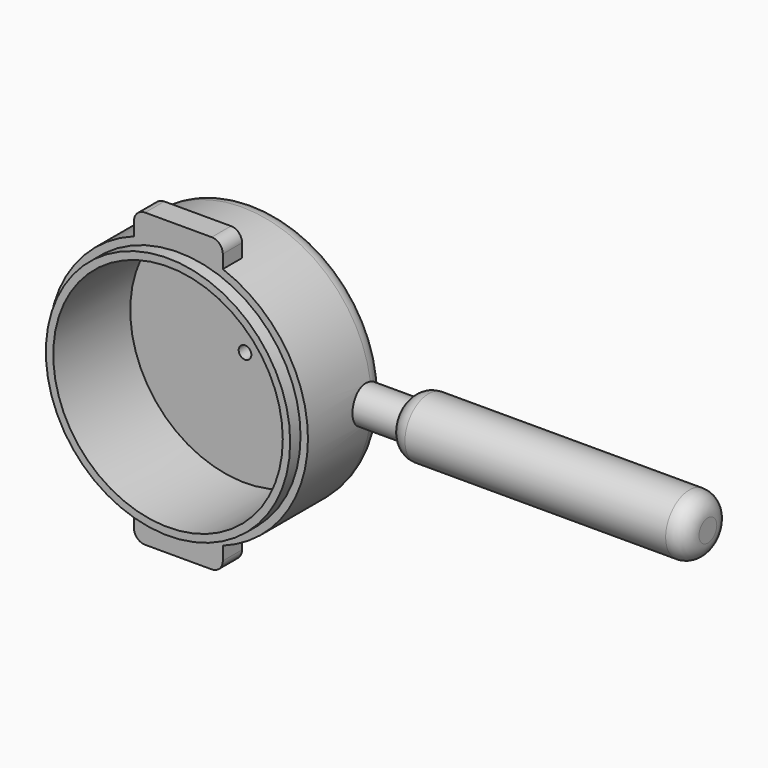
from build123d import *

# Parameters (mm, degrees)
F0_R      = 35
F1_DEPTH  = 30
F2_T      = -4
F3_R      = 5
F5_R      = 5
F7_R      = 8
F7_R_2    = 5
F8_DEPTH  = 80
F9_R      = 5.0065220345
F10_DEPTH = 7
F11_SIZE  = 2
F14_DEPTH = 6.5
F15_R     = 5
F17_R     = 35
F17_R_2   = 33
F18_DEPTH = 3.5
F19_R     = 3
F20_R     = 1.7097163671
F21_DEPTH = 37.001


# Not quite as in the source:
# - a fillet or chamfer that OpenCascade refuses, or shapes differently, is made with other operations: its cross-section is extruded or revolved along the edge and cut away or added


with BuildPart() as f1:
    # F0 (on Front) → F1 (new body)
    with BuildSketch(Plane.XZ):
        Circle(F0_R)
    extrude(amount=F1_DEPTH)

    # F2
    f2_openings = [f1.faces().sort_by_distance(p)[0] for p in [
        (0, -30, 0),
    ]]
    offset(amount=F2_T, openings=f2_openings)

    # F3
    f3_edges = [f1.edges().sort_by_distance(p)[0] for p in [
        (-35, 0, 0),
    ]]
    fillet(f3_edges, radius=F3_R)

    # F5 (on offset) → F6 (join, up to the next surface of F1)
    with BuildSketch(Plane.YZ.offset(47)):
        with Locations((-6.4707305679, 0)):
            Circle(F5_R)
    extrude(until=Until.NEXT, dir=(-1, 0, 0))

    # F7 (on face) → F8 (join)
    with BuildSketch(Plane.YZ.offset(47)):
        with Locations((-6.4707305679, 0)):
            Circle(F7_R)
        with Locations((-6.4707305679, 0)):
            Circle(F7_R_2, mode=Mode.SUBTRACT)
        with Locations((-6.4707305679, 0)):
            Circle(F7_R_2)
    extrude(amount=F8_DEPTH)

    # F9 (on face) → F10 (join)
    with BuildSketch(Plane(origin=(0, 0, 0), x_dir=(-1, 0, 0), z_dir=(0, 1, 0))):
        Circle(F9_R)
    extrude(amount=F10_DEPTH)

    # F11
    f11_edges = [f1.edges().sort_by_distance(p)[0] for p in [
        (5.006522, 7, 0),
    ]]
    chamfer(f11_edges, length=F11_SIZE)

    # F13 (on offset) → F14 (join)
    with BuildSketch(Plane.XZ.offset(26.5)):
        with BuildLine():
            Line((-12, -39.5), (12, -39.5))
            Line((12, -39.5), (12, -32.8785644455))
            ThreePointArc((12, -32.8785644455), (0, -35), (-12, -32.8785644455))
            Line((-12, -32.8785644455), (-12, -39.5))
        make_face()
        with BuildLine():
            ThreePointArc((-12, 32.8785644455), (0, 35), (12, 32.8785644455))
            Line((12, 32.8785644455), (12, 39.5))
            Line((12, 39.5), (-12, 39.5))
            Line((-12, 39.5), (-12, 32.8785644455))
        make_face()
    extrude(amount=-F14_DEPTH)

    # F15
    f15_edges = [f1.edges().sort_by_distance(p)[0] for p in [
        (127, -14.470731, 0),
    ]]
    fillet(f15_edges, radius=F15_R)

    # F16: fillet of radius 5 on 1 edges, made by hand

    # F16_s1 → F16_t2 (revolve, cut)
    with BuildSketch(Plane.XY):
        with BuildLine():
            ThreePointArc((51.582575695, 1.5292694321), (48.8439629074, 0.7125695648), (47, -1.4707305679))
            Line((47, -1.4707305679), (47, 1.5292694321))
            Line((47, 1.5292694321), (51.582575695, 1.5292694321))
        make_face()
    revolve(axis=Axis((47, -6.4707305679, 0), (1, 0, 0)), mode=Mode.SUBTRACT)

    # F17 (on face) → F18 (cut, through all)
    with BuildSketch(Plane.XZ.offset(30)):
        Circle(F17_R)
        Circle(F17_R_2, mode=Mode.SUBTRACT)
    extrude(amount=-F18_DEPTH, mode=Mode.SUBTRACT)

    # F19
    f19_edges = [f1.edges().sort_by_distance(p)[0] for p in [
        (12, -23.25, 39.5),
        (-12, -23.25, 39.5),
        (-12, -23.25, -39.5),
        (12, -23.25, -39.5),
    ]]
    fillet(f19_edges, radius=F19_R)

    # F20 (on face) → F21 (cut, through all)
    with BuildSketch(Plane(origin=(0, 7, 0), x_dir=(-1, 0, 0), z_dir=(0, 1, 0))):
        Circle(F20_R)
    extrude(amount=-F21_DEPTH, mode=Mode.SUBTRACT)


solid = f1.part
